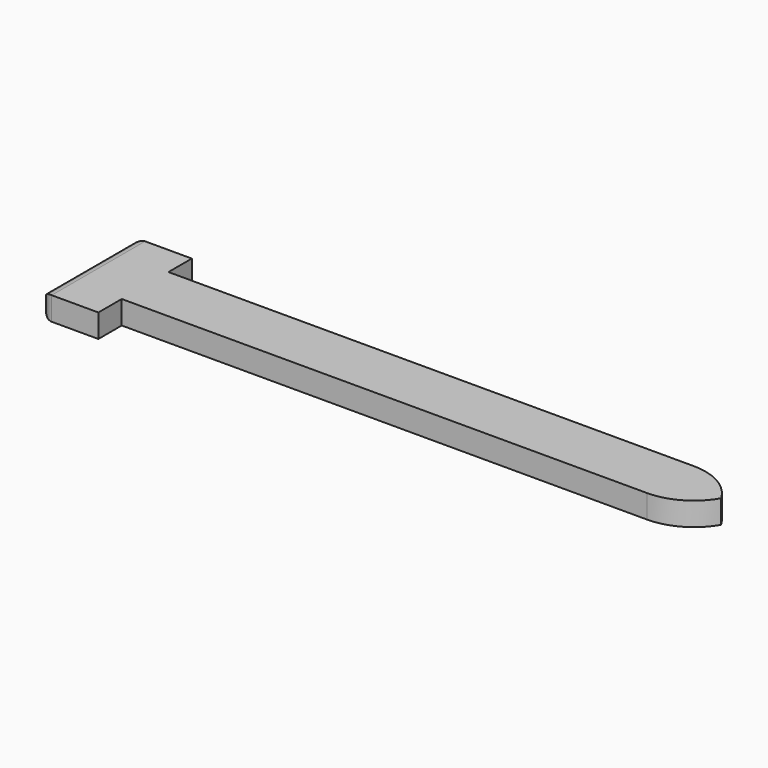
from build123d import *

# Parameters (mm, degrees)
F1_DEPTH    = 2
F2_R        = 0.99999
F3_T1_DEPTH = 27


# Not quite as in the source:
# - a fillet or chamfer that OpenCascade refuses, or shapes differently, is made with other operations: its cross-section is extruded or revolved along the edge and cut away or added
# - a fillet or chamfer is up to 0.001 mm smaller than in the source, because OpenCascade refuses the exact size


with BuildPart() as f1:
    # F0 (on Top) → F1 (new body)
    with BuildSketch(Plane.XY):
        Polygon((-25, 0), (-25, 2.5), (-25, 5), (-30, 5), (-30, -5), (-25, -5), (-25, -2.5), align=None)
        Polygon((25, -2.5), (25, 2.5), (-25, 2.5), (-25, 0), (-25, -2.5), align=None)
    extrude(amount=F1_DEPTH)

    # F2 (radius 1 in the source; OpenCascade refuses exactly that, so slightly less here)
    f2_edges = [f1.edges().sort_by_distance(p)[0] for p in [
        (-30, -5, 1),
        (-30, 0, 2),
        (-30, 5, 1),
        (-30, 0, 0),
    ]]
    fillet(f2_edges, radius=F2_R)

    # F3: fillet of radius 5 on 2 edges, made by hand

    # F3_s2 → F3_t1 (cut)
    with BuildSketch(Plane.XY.offset(-12.5)):
        with BuildLine():
            ThreePointArc((25, 2.5), (23.5355339059, -1.0355339059), (20, -2.5))
            Line((20, -2.5), (25, -2.5))
            Line((25, -2.5), (25, 2.5))
        make_face()
        with BuildLine():
            ThreePointArc((20, 2.5), (23.5355339059, 1.0355339059), (25, -2.5))
            Line((25, -2.5), (25, 2.5))
            Line((25, 2.5), (20, 2.5))
        make_face()
    extrude(amount=F3_T1_DEPTH, mode=Mode.SUBTRACT)


solid = f1.part
